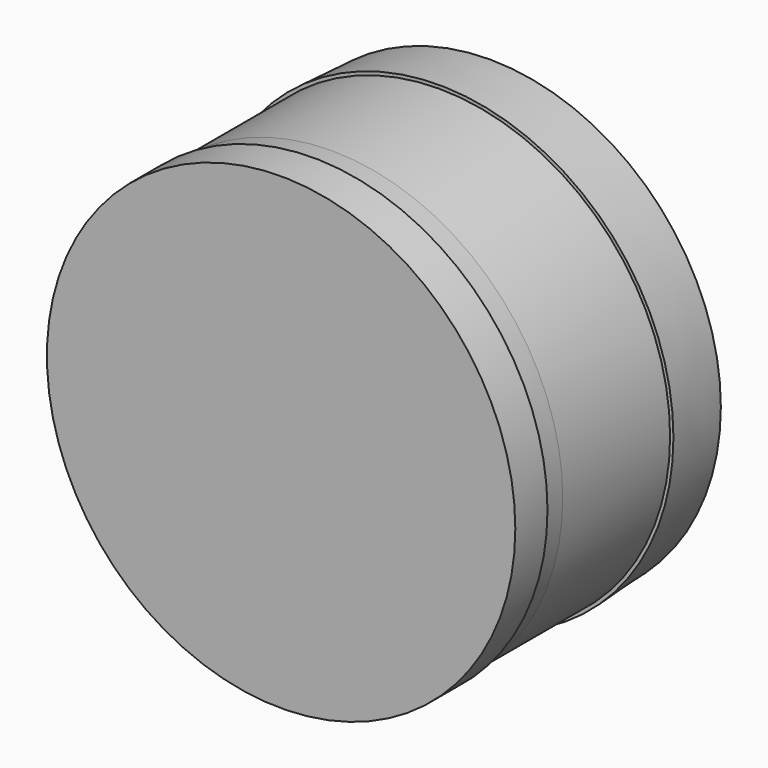
from build123d import *

# Parameters (mm, degrees)
F0_R       = 103.556034567
F1_DEPTH   = 88.646
F1_FACE_R  = 103.556034567
F1_FACE1_R = 103.556034567
F3_DEPTH   = 28.448
F3_TAPER   = -3
F4_DEPTH   = 18.034


# Not quite as in the source:
# - a feature names something its author has since deleted; it is built from what else it names


with BuildPart() as f1:
    # F0 (on Front) → F1 (new body)
    with BuildSketch(Plane.XZ):
        Circle(F0_R)
    extrude(amount=F1_DEPTH)

    # F1_face (on face) + F1_face1 (on face) → F3 (join)
    with BuildSketch(Plane.XZ.offset(88.646)):
        Circle(F1_FACE_R)
    with BuildSketch(Plane(origin=(0, 0, 0), x_dir=(1, 0, 0), z_dir=(0, 1, 0))):
        Circle(F1_FACE1_R)
    extrude(amount=F3_DEPTH, taper=F3_TAPER, dir=(0, -1, 0))

    # F4 (add): a face of the model
    f4_faces = [f1.faces().sort_by_distance(p)[0] for p in [
        (0, -117.094, 0),
    ]]
    extrude(f4_faces, amount=-F4_DEPTH)


solid = f1.part
